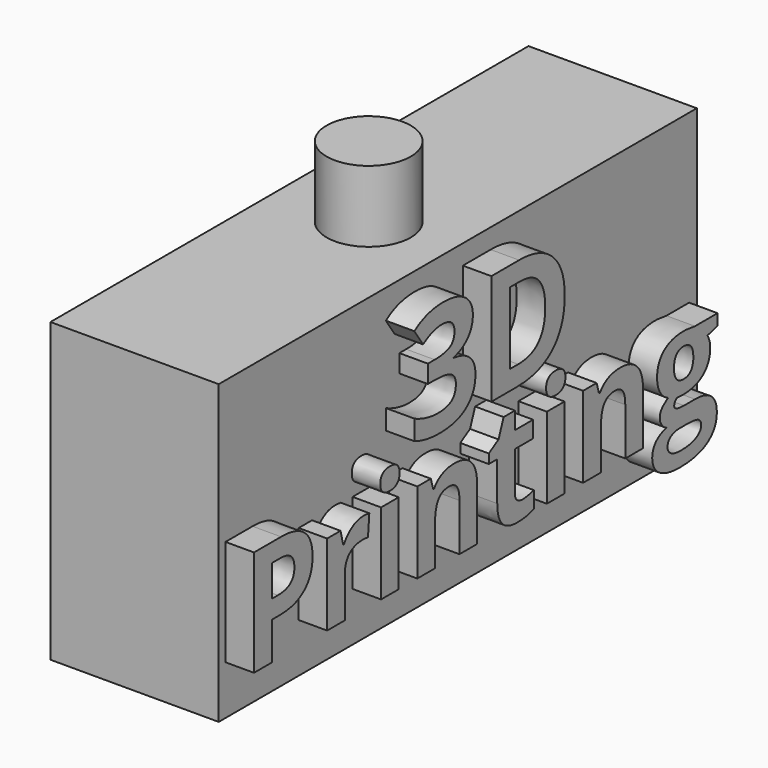
from build123d import *

# Parameters (mm, degrees)
F0_W           = 106.5187280504
F0_H           = 53
F1_DEPTH       = 30
F2_TEXT_SIZE   = 27.5985905638
F2_TEXT_SIZE_2 = 26.4583333333
F3_DEPTH       = 5.08
F4_R           = 7.5
F5_DEPTH       = 12.7


# Not quite as in the source:
# - Text() gives the source's letters only with a copy of the font that has no kerning and outlines rounded to 1/6400 em; it was checked with that copy


with BuildPart() as f1:
    # F0 (on Right) → F1 (new body)
    with BuildSketch(Plane.YZ):
        with Locations((2.0321319101, -38.55718835)):
            Rectangle(F0_W, F0_H)
    extrude(amount=F1_DEPTH)

    # F2 (on face) → F3 (join)
    with BuildSketch(Plane.YZ.offset(30)):
        with Locations((-15.0624886708, -35.2688521692)):
            Text('3D', F2_TEXT_SIZE, font='Open Sans', font_style=FontStyle.BOLD, text_align=(TextAlign.LEFT, TextAlign.BOTTOM))
        with Locations((-52.1003985959, -56.3090160203)):
            Text('Printing', F2_TEXT_SIZE_2, font='Open Sans', font_style=FontStyle.BOLD, text_align=(TextAlign.LEFT, TextAlign.BOTTOM))
    extrude(amount=F3_DEPTH)

    # F4 (on face) → F5 (join)
    with BuildSketch(Plane.XY.offset(-12.05718835)):
        with Locations((15.7503771717, 0)):
            Circle(F4_R)
    extrude(amount=F5_DEPTH)


solid = f1.part
